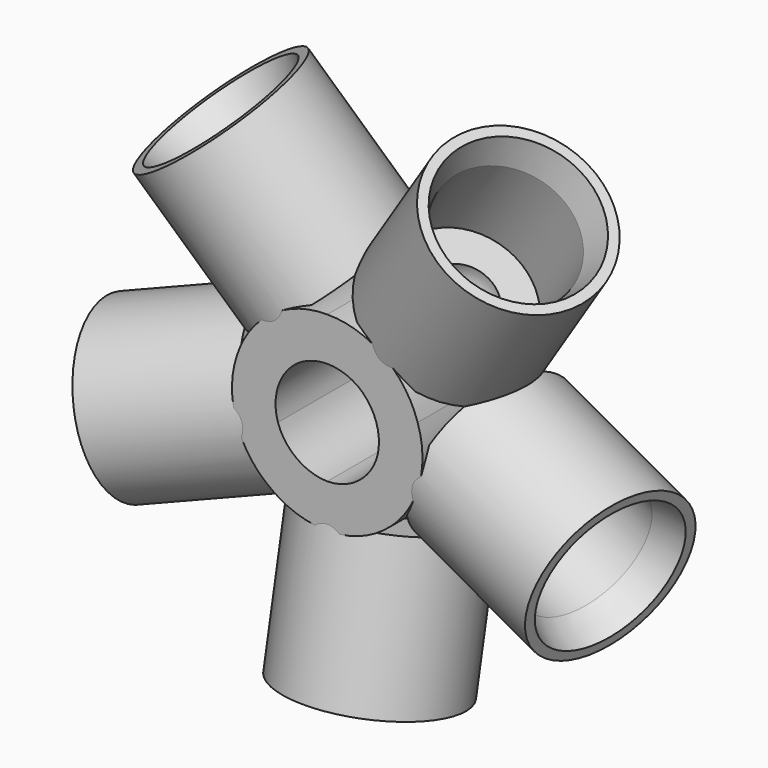
from build123d import *

# Parameters (mm, degrees)
F0_R          = 19.5
F0_R_2        = 11
F4_DEPTH      = 17
F4_DEPTH_BACK = 4
F6_COUNT      = 5
F0_TEXT_SIZE  = 10.7933353219
F7_DEPTH      = 5


# Not quite as in the source:
# - Text() gives the source's letters only with a copy of the font that has no kerning and outlines rounded to 1/6400 em; it was checked with that copy


with BuildPart() as f3:
    # F2 (on line) → F3 (revolve)
    with BuildSketch(Plane(origin=(0, -3.7526447404, 0.7464474492), x_dir=(1, 0, 0), z_dir=(0, -0.9807852804, 0.195090322))):
        with BuildLine():
            Line((6.7275495715, 16.1909703114), (13.39, 16.1909703114))
            Line((13.39, 16.1909703114), (13.39, -5.2532064901))
            Line((13.39, -5.2532064901), (15.39, -11.5995957263))
            Line((15.39, -11.5995957263), (17.39, -11.5995957263))
            Line((17.39, -11.5995957263), (17.39, 20.1909703114))
            Line((17.39, 20.1909703114), (8.4690514833, 20.1909703114))
            ThreePointArc((8.4690514833, 20.1909703114), (5.0129940493, 24.1026530457), (0, 25.557123899))
            Line((0, 25.557123899), (0, 22.9185198829))
            ThreePointArc((0, 22.9185198829), (4.7570959228, 20.9480662342), (6.7275495715, 16.1909703114))
        make_face()
    revolve(axis=Axis((0, 0.9759197373, 24.5185463889), (0, 0.195090322, 0.9807852804)))

    # F0 (on Front) → F4 (join, two sides)
    with BuildSketch(Plane.XZ) as f4_sk:
        with Locations((0, 41.6122665526)):
            Circle(F0_R)
        with Locations((0, 41.6122665526)):
            Circle(F0_R_2, mode=Mode.SUBTRACT)
        with BuildLine():
            Line((11.9458946412, 38.7280322611), (11.9458946412, 46.4334618058))
            Line((11.9458946412, 46.4334618058), (14.1231127507, 46.4334618058))
            add(Edge.make_bspline(
                [(14.1231127507, 46.4334618058), (15.6561036581, 46.4334618058), (16.3416490969, 45.9747450546)],
                knots=[0, 0, 0, 1, 1, 1], degree=2))
            add(Edge.make_bspline(
                [(16.3416490969, 45.9747450546), (17.0271945357, 45.5160283034), (17.0271945357, 44.5260770794)],
                knots=[0, 0, 0, 1, 1, 1], degree=2))
            add(Edge.make_bspline(
                [(17.0271945357, 44.5260770794), (17.0271945357, 43.8396884112), (16.6452116529, 43.3944633292)],
                knots=[0, 0, 0, 1, 1, 1], degree=2))
            add(Edge.make_bspline(
                [(16.6452116529, 43.3944633292), (16.26322877, 42.9492382472), (15.5296192598, 42.8176944729)],
                knots=[0, 0, 0, 1, 1, 1], degree=2))
            Line((15.5296192598, 42.8176944729), (15.5296192598, 42.765414255))
            add(Edge.make_bspline(
                [(15.5296192598, 42.765414255), (17.2852227083, 42.4652246163), (17.2852227083, 40.9204284984)],
                knots=[0, 0, 0, 1, 1, 1], degree=2))
            add(Edge.make_bspline(
                [(17.2852227083, 40.9204284984), (17.2852227083, 39.8883158082), (16.5870288296, 39.3081740347)],
                knots=[0, 0, 0, 1, 1, 1], degree=2))
            add(Edge.make_bspline(
                [(16.5870288296, 39.3081740347), (15.888834951, 38.7280322611), (14.6341097198, 38.7280322611)],
                knots=[0, 0, 0, 1, 1, 1], degree=2))
            Line((14.6341097198, 38.7280322611), (11.9458946412, 38.7280322611))
        make_face(mode=Mode.SUBTRACT)
    extrude(amount=F4_DEPTH)
    extrude(f4_sk.sketch, amount=-F4_DEPTH_BACK)


with BuildPart() as f6_1:
    # F6: instance of F3
    add(f3.part.rotate(Axis((0, -4.9195094034, 41.8967977166), (0, 1, 0)), 1 * 360 / F6_COUNT))


with BuildPart() as f6_2:
    # F6: instance of F3
    add(f3.part.rotate(Axis((0, -4.9195094034, 41.8967977166), (0, 1, 0)), 2 * 360 / F6_COUNT))


with BuildPart() as f6_3:
    # F6: instance of F3
    add(f3.part.rotate(Axis((0, -4.9195094034, 41.8967977166), (0, 1, 0)), 3 * 360 / F6_COUNT))


with BuildPart() as f6_4:
    # F6: instance of F3
    add(f3.part.rotate(Axis((0, -4.9195094034, 41.8967977166), (0, 1, 0)), 4 * 360 / F6_COUNT))


with BuildPart() as f3_1:
    add(f3.part)

    add(f6_1.part)  # F7 merges F6_1

    add(f6_2.part)  # F7 merges F6_2

    add(f6_3.part)  # F7 merges F6_3

    add(f6_4.part)  # F7 merges F6_4
    # F0 (on Front) → F7 (join)
    with BuildSketch(Plane.XZ):
        with Locations((10.8867986128, 38.7280322611)):
            Text('B', F0_TEXT_SIZE, font='Open Sans', text_align=(TextAlign.LEFT, TextAlign.BOTTOM))
    extrude(amount=-F7_DEPTH)


solid = f3_1.part
